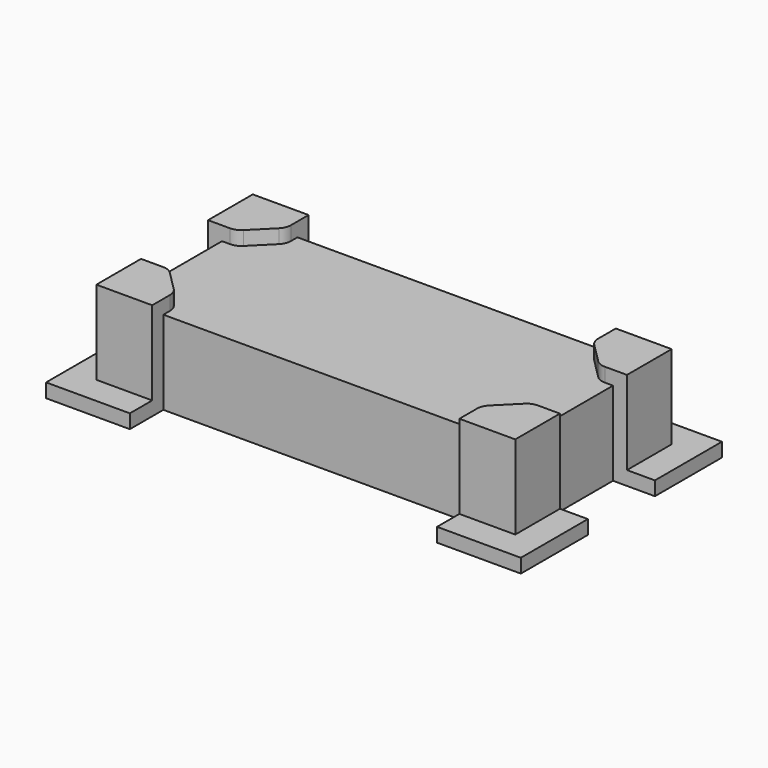
from build123d import *

# Parameters (mm, degrees)
F0_W     = 177.8
F0_H     = 76.2
F1_DEPTH = 38.1
F3_DEPTH = 38.1
F5_DEPTH = 6.35
F6_DEPTH = 6.35


with BuildPart() as f1:
    # F0 (on Top) → F1 (new body)
    with BuildSketch(Plane.XY):
        Rectangle(F0_W, F0_H)
    extrude(amount=F1_DEPTH)


with BuildPart() as f3:
    # F2 (on Top) → F3 (new body, through all)
    with BuildSketch(Plane.XY):
        Polygon((-69.85, -38.1), (-88.9, -38.1), (-88.9, -19.05), (-95.25, -19.05), (-95.25, -44.45), (-69.85, -44.45), align=None)
        with BuildLine():
            Line((-88.9, -19.05), (-88.9, -38.1))
            Line((-88.9, -38.1), (-69.85, -38.1))
            Line((-69.85, -38.1), (-69.85, -34.3802561211))
            ThreePointArc((-69.85, -34.3802561211), (-70.3333649686, -31.9502163256), (-71.7098719395, -29.8901280605))
            Line((-71.7098719395, -29.8901280605), (-80.6901280605, -20.9098719395))
            ThreePointArc((-80.6901280605, -20.9098719395), (-82.7502163256, -19.5333649686), (-85.1802561211, -19.05))
            Line((-85.1802561211, -19.05), (-88.9, -19.05))
        make_face()
    extrude(amount=F3_DEPTH)

    # F4 (on face) → F5 (join)
    with BuildSketch(Plane.XY.offset(38.1)):
        with BuildLine():
            Line((-88.9, -38.1), (-69.85, -38.1))
            Line((-69.85, -38.1), (-69.85, -34.3802561211))
            ThreePointArc((-69.85, -34.3802561211), (-70.3333649686, -31.9502163256), (-71.7098719395, -29.8901280605))
            Line((-71.7098719395, -29.8901280605), (-80.6901280605, -20.9098719395))
            ThreePointArc((-80.6901280605, -20.9098719395), (-82.7502163256, -19.5333649686), (-85.1802561211, -19.05))
            Line((-85.1802561211, -19.05), (-88.9, -19.05))
            Line((-88.9, -19.05), (-88.9, -38.1))
        make_face()
        Polygon((-69.85, -44.45), (-69.85, -38.1), (-88.9, -38.1), (-88.9, -19.05), (-95.25, -19.05), (-95.25, -44.45), align=None)
    extrude(amount=F5_DEPTH)

    # F2 (on Top) → F6, piece 4 (join)
    with BuildSketch(Plane.XY):
        Polygon((-69.85, -57.15), (-69.85, -44.45), (-95.25, -44.45), (-95.25, -19.05), (-107.95, -19.05), (-107.95, -57.15), align=None)
    extrude(amount=F6_DEPTH)


with BuildPart() as f3b:
    # F2 (on Top) → F3, piece 2 (new body, through all)
    with BuildSketch(Plane.XY):
        with BuildLine():
            Line((-88.9, 38.1), (-88.9, 19.05))
            Line((-88.9, 19.05), (-85.1802561211, 19.05))
            ThreePointArc((-85.1802561211, 19.05), (-82.7502163256, 19.5333649686), (-80.6901280605, 20.9098719395))
            Line((-80.6901280605, 20.9098719395), (-71.7098719395, 29.8901280605))
            ThreePointArc((-71.7098719395, 29.8901280605), (-70.3333649686, 31.9502163256), (-69.85, 34.3802561211))
            Line((-69.85, 34.3802561211), (-69.85, 38.1))
            Line((-69.85, 38.1), (-88.9, 38.1))
        make_face()
        Polygon((-95.25, 19.05), (-88.9, 19.05), (-88.9, 38.1), (-69.85, 38.1), (-69.85, 44.45), (-95.25, 44.45), align=None)
    extrude(amount=F3_DEPTH)

    # F4 (on face) → F5, piece 2 (join)
    with BuildSketch(Plane.XY.offset(38.1)):
        with BuildLine():
            ThreePointArc((-71.7098719395, 29.8901280605), (-70.3333649686, 31.9502163256), (-69.85, 34.3802561211))
            Line((-69.85, 34.3802561211), (-69.85, 38.1))
            Line((-69.85, 38.1), (-88.9, 38.1))
            Line((-88.9, 38.1), (-88.9, 19.05))
            Line((-88.9, 19.05), (-85.1802561211, 19.05))
            ThreePointArc((-85.1802561211, 19.05), (-82.7502163256, 19.5333649686), (-80.6901280605, 20.9098719395))
            Line((-80.6901280605, 20.9098719395), (-71.7098719395, 29.8901280605))
        make_face()
        Polygon((-88.9, 38.1), (-69.85, 38.1), (-69.85, 44.45), (-95.25, 44.45), (-95.25, 19.05), (-88.9, 19.05), align=None)
    extrude(amount=F5_DEPTH)

    # F2 (on Top) → F6, piece 2 (join)
    with BuildSketch(Plane.XY):
        Polygon((-107.95, 19.05), (-95.25, 19.05), (-95.25, 44.45), (-69.85, 44.45), (-69.85, 57.15), (-107.95, 57.15), align=None)
    extrude(amount=F6_DEPTH)


with BuildPart() as f3c:
    # F2 (on Top) → F3, piece 3 (new body, through all)
    with BuildSketch(Plane.XY):
        with BuildLine():
            Line((69.85, -34.3802561211), (69.85, -38.1))
            Line((69.85, -38.1), (88.9, -38.1))
            Line((88.9, -38.1), (88.9, -19.05))
            Line((88.9, -19.05), (85.1802561211, -19.05))
            ThreePointArc((85.1802561211, -19.05), (82.7502163256, -19.5333649686), (80.6901280605, -20.9098719395))
            Line((80.6901280605, -20.9098719395), (71.7098719395, -29.8901280605))
            ThreePointArc((71.7098719395, -29.8901280605), (70.3333649686, -31.9502163256), (69.85, -34.3802561211))
        make_face()
        Polygon((88.9, -38.1), (69.85, -38.1), (69.85, -44.45), (95.25, -44.45), (95.25, -19.05), (88.9, -19.05), align=None)
    extrude(amount=F3_DEPTH)

    # F4 (on face) → F5, piece 3 (join)
    with BuildSketch(Plane.XY.offset(38.1)):
        with BuildLine():
            Line((88.9, -38.1), (88.9, -19.05))
            Line((88.9, -19.05), (85.1802561211, -19.05))
            ThreePointArc((85.1802561211, -19.05), (82.7502163256, -19.5333649686), (80.6901280605, -20.9098719395))
            Line((80.6901280605, -20.9098719395), (71.7098719395, -29.8901280605))
            ThreePointArc((71.7098719395, -29.8901280605), (70.3333649686, -31.9502163256), (69.85, -34.3802561211))
            Line((69.85, -34.3802561211), (69.85, -38.1))
            Line((69.85, -38.1), (88.9, -38.1))
        make_face()
        Polygon((95.25, -19.05), (88.9, -19.05), (88.9, -38.1), (69.85, -38.1), (69.85, -44.45), (95.25, -44.45), align=None)
    extrude(amount=F5_DEPTH)

    # F2 (on Top) → F6, piece 3 (join)
    with BuildSketch(Plane.XY):
        Polygon((95.25, -44.45), (69.85, -44.45), (69.85, -57.15), (107.95, -57.15), (107.95, -19.05), (95.25, -19.05), align=None)
    extrude(amount=F6_DEPTH)


with BuildPart() as f3d:
    # F2 (on Top) → F3, piece 4 (new body, through all)
    with BuildSketch(Plane.XY):
        with BuildLine():
            Line((85.1802561211, 19.05), (88.9, 19.05))
            Line((88.9, 19.05), (88.9, 38.1))
            Line((88.9, 38.1), (69.85, 38.1))
            Line((69.85, 38.1), (69.85, 34.3802561211))
            ThreePointArc((69.85, 34.3802561211), (70.3333649686, 31.9502163256), (71.7098719395, 29.8901280605))
            Line((71.7098719395, 29.8901280605), (80.6901280605, 20.9098719395))
            ThreePointArc((80.6901280605, 20.9098719395), (82.7502163256, 19.5333649686), (85.1802561211, 19.05))
        make_face()
        Polygon((88.9, 38.1), (88.9, 19.05), (95.25, 19.05), (95.25, 44.45), (69.85, 44.45), (69.85, 38.1), align=None)
    extrude(amount=F3_DEPTH)

    # F4 (on face) → F5, piece 4 (join)
    with BuildSketch(Plane.XY.offset(38.1)):
        with BuildLine():
            Line((71.7098719395, 29.8901280605), (80.6901280605, 20.9098719395))
            ThreePointArc((80.6901280605, 20.9098719395), (82.7502163256, 19.5333649686), (85.1802561211, 19.05))
            Line((85.1802561211, 19.05), (88.9, 19.05))
            Line((88.9, 19.05), (88.9, 38.1))
            Line((88.9, 38.1), (69.85, 38.1))
            Line((69.85, 38.1), (69.85, 34.3802561211))
            ThreePointArc((69.85, 34.3802561211), (70.3333649686, 31.9502163256), (71.7098719395, 29.8901280605))
        make_face()
        Polygon((88.9, 38.1), (88.9, 19.05), (95.25, 19.05), (95.25, 44.45), (69.85, 44.45), (69.85, 38.1), align=None)
    extrude(amount=F5_DEPTH)

    # F2 (on Top) → F6 (join)
    with BuildSketch(Plane.XY):
        Polygon((95.25, 44.45), (95.25, 19.05), (107.95, 19.05), (107.95, 57.15), (69.85, 57.15), (69.85, 44.45), align=None)
    extrude(amount=F6_DEPTH)


solid = Compound([f1.part, f3.part, f3b.part, f3c.part, f3d.part])
